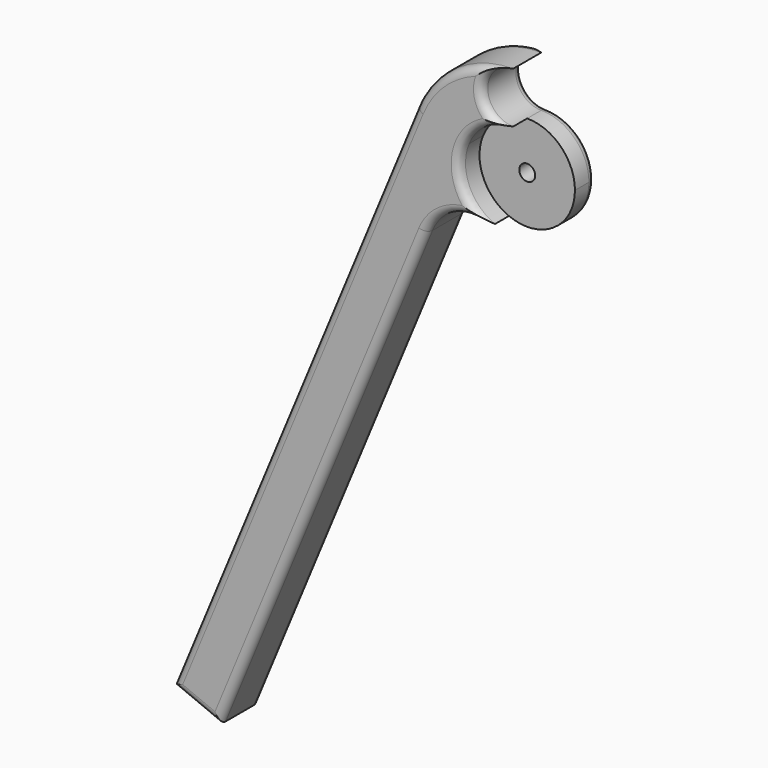
from build123d import *

# Parameters (mm, degrees)
F1_DEPTH     = 16
F2_DEPTH     = 8
F3_T1_DEPTH  = 28.5
F3_T3_DEPTH  = 176.25
F3_T5_DEPTH  = 206.25
F3_T8_ANGLE  = 113.8828315396
F3_T10_ANGLE = 205.3052563157
F3_T12_ANGLE = 301.0526480562
F3_T14_ANGLE = 87.1421031631
F3_T16_ANGLE = 90
F3_T18_ANGLE = 202.4999999088
F3_T20_ANGLE = 256.2183340246
F3_T22_ANGLE = 87.1421031631
F4_D         = 5


# Not quite as in the source:
# - a fillet or chamfer that OpenCascade refuses, or shapes differently, is made with other operations: its cross-section is extruded or revolved along the edge and cut away or added


with BuildPart() as f1:
    # F0 (on Front) → F1 (new body)
    with BuildSketch(Plane.XZ):
        Polygon((-25.3386959586, -21.9761344899), (-13.8581929877, 5.7402514855), (-28.6402655078, 11.8631864033), (-105.1769519809, -172.9127200989), (-90.3948794607, -179.0356550168), align=None)
        with BuildLine():
            Line((-28.6402655078, 11.8631864033), (-13.8581929877, 5.7402514855))
            ThreePointArc((-13.8581929877, 5.7402514855), (-8.3335534854, 12.4720441912), (2.39e-08, 15))
            ThreePointArc((2.39e-08, 15), (-8, 22.9999999881), (0, 31))
            ThreePointArc((0, 31), (-17.2226772236, 25.7755579814), (-28.6402655078, 11.8631864033))
        make_face()
        with BuildLine():
            ThreePointArc((-5.7402514855, -13.8581929877), (-13.8581929877, -5.7402514855), (-13.8581929877, 5.7402514855))
            Line((-13.8581929877, 5.7402514855), (-25.3386959586, -21.9761344899))
            ThreePointArc((-25.3386959586, -21.9761344899), (-17.2207544564, -13.8581929877), (-5.7402514855, -13.8581929877))
        make_face()
    extrude(amount=F1_DEPTH)

    # F0 (on Front) → F2 (join)
    with BuildSketch(Plane.XZ):
        with BuildLine():
            Line((0, 0), (-13.8581929877, 5.7402514855))
            ThreePointArc((-13.8581929877, 5.7402514855), (-13.8581929877, -5.7402514855), (-5.7402514855, -13.8581929877))
            Line((-5.7402514855, -13.8581929877), (0, 0))
        make_face()
        with BuildLine():
            ThreePointArc((2.39e-08, 15), (-8.3335534854, 12.4720441912), (-13.8581929877, 5.7402514855))
            Line((-13.8581929877, 5.7402514855), (0, 0))
            Line((0, 0), (-5.7402514855, -13.8581929877))
            ThreePointArc((-5.7402514855, -13.8581929877), (8.3335534953, -12.4720441845), (15, 0))
            ThreePointArc((15, 0), (10.6066017262, 10.6066017094), (2.39e-08, 15))
        make_face()
    extrude(amount=F2_DEPTH)

    # F3: fillet of radius 2.5 on 14 edges, made by hand

    # F3_s2 → F3_t1 (cut)
    with BuildSketch(Plane(origin=(-34.414512586, 0, 14.2549578556), x_dir=(0, 1, 0), z_dir=(0.9238795325, 0, -0.3826834324))):
        with BuildLine():
            ThreePointArc((-13.5, -200), (-15.267766953, -199.267766953), (-16, -197.5))
            Line((-16, -197.5), (-16, -200))
            Line((-16, -200), (-13.5, -200))
        make_face()
        with BuildLine():
            ThreePointArc((-2.5, -200), (-0.732233047, -199.267766953), (0, -197.5))
            Line((0, -197.5), (0, -200))
            Line((0, -200), (-2.5, -200))
        make_face()
    extrude(amount=F3_T1_DEPTH, mode=Mode.SUBTRACT)

    # F3_s4 → F3_t3 (cut)
    with BuildSketch(Plane(origin=(-78.9284579253, 0, -190.5501535805), x_dir=(0, 1, 0), z_dir=(0.3826834324, 0, 0.9238795325))):
        with BuildLine():
            ThreePointArc((-13.5, 15), (-15.267766953, 15.732233047), (-16, 17.5))
            Line((-16, 17.5), (-16, 15))
            Line((-16, 15), (-13.5, 15))
        make_face()
        with BuildLine():
            ThreePointArc((-2.5, 15), (-0.732233047, 15.732233047), (0, 17.5))
            Line((0, 17.5), (0, 15))
            Line((0, 15), (-2.5, 15))
        make_face()
    extrude(amount=F3_T3_DEPTH, mode=Mode.SUBTRACT)

    # F3_s6 → F3_t5 (cut)
    with BuildSketch(Plane(origin=(0, 0, 0), x_dir=(0, 1, 0), z_dir=(-0.3826834324, 0, -0.9238795325))):
        with BuildLine():
            ThreePointArc((-13.5, -31), (-15.267766953, -30.267766953), (-16, -28.5))
            Line((-16, -28.5), (-16, -31))
            Line((-16, -31), (-13.5, -31))
        make_face()
        with BuildLine():
            ThreePointArc((-2.5, -31), (-0.732233047, -30.267766953), (0, -28.5))
            Line((0, -28.5), (0, -31))
            Line((0, -31), (-2.5, -31))
        make_face()
    extrude(amount=F3_T5_DEPTH, mode=Mode.SUBTRACT)

    # F3_s7 → F3_t8 (revolve, cut)
    with BuildSketch(Plane(origin=(-11.480502971, 0, -27.7163859753), x_dir=(0, 1, 0), z_dir=(-0.3826834324, 0, -0.9238795325))):
        with BuildLine():
            ThreePointArc((-16, -17.5), (-15.267766953, -15.732233047), (-13.5, -15))
            Line((-13.5, -15), (-16, -15))
            Line((-16, -15), (-16, -17.5))
        make_face()
    revolve(axis=Axis((-11.480502971, -16, -27.7163859753), (0, 1, 0)), revolution_arc=F3_T8_ANGLE, mode=Mode.SUBTRACT)

    # F3_s9 → F3_t10 (revolve, cut)
    with BuildSketch(Plane(origin=(0, 0, 0), x_dir=(0, 1, 0), z_dir=(0.999700368, 0, 0.0244780336))):
        with BuildLine():
            ThreePointArc((-16, -17.5), (-15.267766953, -15.732233047), (-13.5, -15))
            Line((-13.5, -15), (-16, -15))
            Line((-16, -15), (-16, -17.5))
        make_face()
    revolve(axis=Axis((0, -16, 0), (0, 1, 0)), revolution_arc=F3_T10_ANGLE, mode=Mode.SUBTRACT)

    # F3_s11 → F3_t12 (revolve, cut)
    with BuildSketch(Plane(origin=(11.4998076678, 0, 11.4334898289), x_dir=(0, 1, 0), z_dir=(0.7091486068, 0, 0.7050590425))):
        with BuildLine():
            ThreePointArc((-16, 5.8104179571), (-15.267766953, 7.5781849101), (-13.5, 8.3104179571))
            Line((-13.5, 8.3104179571), (-16, 8.3104179571))
            Line((-16, 8.3104179571), (-16, 5.8104179571))
        make_face()
    revolve(axis=Axis((0, -16, 23), (0, 1, 0)), revolution_arc=F3_T12_ANGLE, mode=Mode.SUBTRACT)

    # F3_s13 → F3_t14 (revolve, cut)
    with BuildSketch(Plane(origin=(0, 0, 0), x_dir=(0, 1, 0), z_dir=(0.9418106956, 0, -0.3361437395))):
        with BuildLine():
            ThreePointArc((-16, 28.5), (-15.267766953, 30.267766953), (-13.5, 31))
            Line((-13.5, 31), (-16, 31))
            Line((-16, 31), (-16, 28.5))
        make_face()
    revolve(axis=Axis((0, -16, 0), (0, -1, 0)), revolution_arc=F3_T14_ANGLE, mode=Mode.SUBTRACT)

    # F3_s15 → F3_t16 (revolve, cut)
    with BuildSketch(Plane(origin=(-11.480502971, 0, -27.7163859753), x_dir=(0, 1, 0), z_dir=(-0.3826834324, 0, -0.9238795325))):
        with BuildLine():
            ThreePointArc((0, -17.5), (-0.732233047, -15.732233047), (-2.5, -15))
            Line((-2.5, -15), (0, -15))
            Line((0, -15), (0, -17.5))
        make_face()
    revolve(axis=Axis((-11.480502971, 0, -27.7163859753), (0, 1, 0)), revolution_arc=F3_T16_ANGLE, mode=Mode.SUBTRACT)

    # F3_s17 → F3_t18 (revolve, cut)
    with BuildSketch(Plane(origin=(0, 0, 0), x_dir=(0, 1, 0), z_dir=(-0.9238795325, 0, 0.3826834324))):
        with BuildLine():
            ThreePointArc((0, 12.5), (-0.732233047, 14.267766953), (-2.5, 15))
            Line((-2.5, 15), (0, 15))
            Line((0, 15), (0, 12.5))
        make_face()
    revolve(axis=Axis((0, 0, 0), (0, -1, 0)), revolution_arc=F3_T18_ANGLE, mode=Mode.SUBTRACT)

    # F3_s19 → F3_t20 (revolve, cut)
    with BuildSketch(Plane.YZ):
        with BuildLine():
            ThreePointArc((0, 12.5), (-0.732233047, 14.267766953), (-2.5, 15))
            Line((-2.5, 15), (0, 15))
            Line((0, 15), (0, 12.5))
        make_face()
    revolve(axis=Axis((0, 0, 23), (0, 1, 0)), revolution_arc=F3_T20_ANGLE, mode=Mode.SUBTRACT)

    # F3_s21 → F3_t22 (revolve, cut)
    with BuildSketch(Plane(origin=(0, 0, 0), x_dir=(0, 1, 0), z_dir=(0.9418106956, 0, -0.3361437395))):
        with BuildLine():
            ThreePointArc((0, 28.5), (-0.732233047, 30.267766953), (-2.5, 31))
            Line((-2.5, 31), (0, 31))
            Line((0, 31), (0, 28.5))
        make_face()
    revolve(axis=Axis((0, 0, 0), (0, -1, 0)), revolution_arc=F3_T22_ANGLE, mode=Mode.SUBTRACT)

    # F4 (through all)
    with Locations(Plane(origin=(0, 0, 0), x_dir=(1, 0, 0), z_dir=(0, 1, 0))):
        with Locations((0, 0)):
            Hole(F4_D / 2)


solid = f1.part
